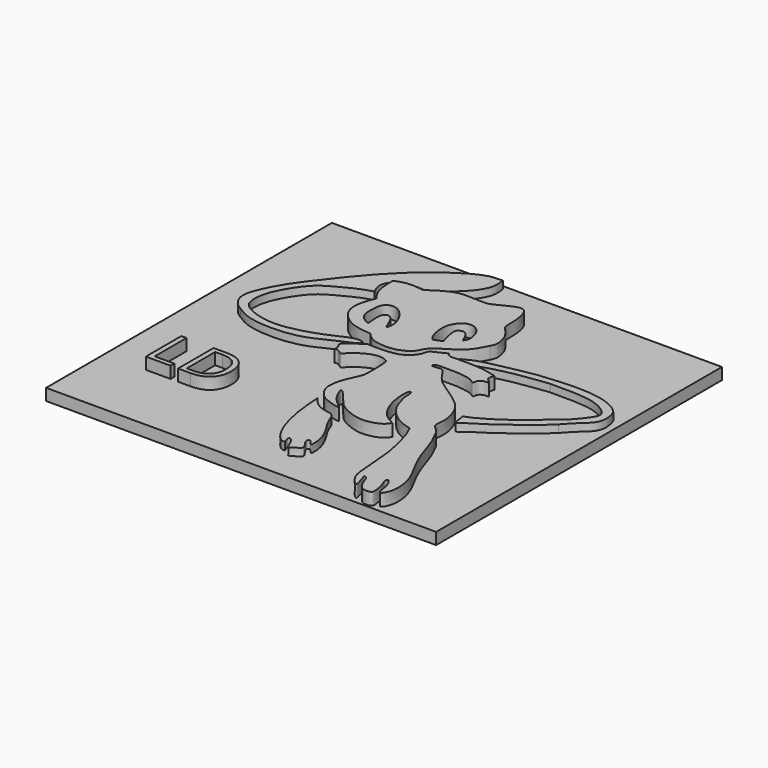
from build123d import *

# Parameters (mm, degrees)
F1_DEPTH     = 5.334
F2_DEPTH     = 3.302
F3_W         = 169.9430719018
F3_H         = 155.6462794542
F4_DEPTH     = 5.08
F5_DEPTH     = 5.08
F6_TEXT_SIZE = 27.0730789958
F7_DEPTH     = 5.08
F8_DEPTH     = 2.54


# Not quite as in the source:
# - Text() gives the source's letters only with a copy of the font that has no kerning and outlines rounded to 1/6400 em; it was checked with that copy


with BuildPart() as f1:
    # F0 (on Top) → F1 (new body)
    with BuildSketch(Plane.XY):
        with BuildLine():
            add(Edge.make_bspline(
                [(-36.8846021593, 36.0807068646), (-37.3919205691, 36.745355779), (-38.573167318, 38.2929329101), (-40.5014475338, 42.4143572996), (-40.7107590613, 48.2182279222), (-40.6138391704, 49.4369952817), (-40.5808985233, 49.8512238264)],
                knots=[0, 0, 0, 0, 0.2194056509, 0.5108669562, 0.8337559114, 1, 1, 1, 1], degree=3))
            add(Edge.make_bspline(
                [(-22.3644245416, 14.6438442171), (-24.6713467296, 14.8439032159), (-29.1783533156, 15.2347561151), (-34.882181479, 17.9727219406), (-39.1312315637, 23.0647945356), (-39.4935763136, 28.8302862551), (-37.8267011281, 33.815991482), (-37.1553457104, 35.4298653868), (-36.8846021593, 36.0807068646)],
                knots=[0, 0, 0, 0, 0.1893684443, 0.3699668893, 0.5515158216, 0.7238806595, 0.8886468645, 1, 1, 1, 1], degree=3))
            add(Edge.make_bspline(
                [(-5.2082133479, 12.2014991939), (-6.1207744444, 11.7172463933), (-8.3286563669, 10.545628396), (-15.353587418, 10.2966075507), (-19.699613734, 11.8971410348), (-21.5102479887, 13.7634179409), (-22.3644245416, 14.6438442171)],
                knots=[0, 0, 0, 0, 0.2165971456, 0.5240426358, 0.775464526, 1, 1, 1, 1], degree=3))
            add(Edge.make_bspline(
                [(15.1303568855, 32.9696908593), (14.5352451306, 31.8316959723), (13.2486953483, 29.3715075085), (10.2455123386, 24.8910940387), (3.5467707647, 21.2909451139), (-0.1632139181, 18.6569829706), (-1.6228436975, 15.6766034686), (-3.1877963332, 12.9531999529), (-4.5795045255, 12.4354117454), (-5.2082133479, 12.2014991939)],
                knots=[0, 0, 0, 0, 0.1407144931, 0.3042053849, 0.4994170574, 0.6491627195, 0.7763538673, 0.8989671128, 1, 1, 1, 1], degree=3))
            add(Edge.make_bspline(
                [(-28.5498145968, 50.8658960462), (-27.3946017427, 51.6630685406), (-24.9466228795, 53.3523342114), (-20.0833499164, 56.0652919109), (-16.3542778469, 56.9634408184), (-12.2867311767, 56.8716252918), (-6.9153223537, 56.7342359886), (-4.3946916269, 56.665054576), (1.0627636823, 59.6982249817), (4.5886739884, 61.236413898), (8.2470343675, 61.4891197316), (9.8575595266, 56.0097175618), (10.1904654801, 52.4142595185), (10.0843781414, 47.0754303269), (11.5893851176, 45.8127835913), (14.8613176101, 41.8496715208), (15.5576528197, 39.0147495294), (16.4135900587, 35.7580508966), (15.5545549064, 33.8914382347), (15.1303568855, 32.9696908593)],
                knots=[0, 0, 0, 0, 0.0621112649, 0.1316182234, 0.188871196, 0.2491962953, 0.3167553376, 0.3643401957, 0.436758445, 0.4967888689, 0.546791506, 0.6123099758, 0.6728165948, 0.7378250462, 0.7790399568, 0.8445049968, 0.8965058511, 0.9488938107, 1, 1, 1, 1], degree=3))
            add(Edge.make_bspline(
                [(-40.5808985233, 49.8512238264), (-39.7577733728, 50.1889108848), (-38.0437485114, 50.8920895121), (-34.9342862767, 51.5058179945), (-31.3792002355, 51.3783823788), (-29.458277106, 51.0304457679), (-28.5498145968, 50.8658960462)],
                knots=[0, 0, 0, 0, 0.234957575, 0.4892611102, 0.7584561682, 1, 1, 1, 1], degree=3))
        make_face()
        with BuildLine():
            add(Edge.make_bspline(
                [(-27.7441535145, 20.2597975731), (-27.836523165, 21.3377254697), (-28.0205851584, 23.4856772729), (-28.2064858053, 26.7533419634), (-27.3095138698, 28.5803581568), (-25.8242693753, 29.158776732), (-23.9397520395, 27.8647529376), (-22.7818146955, 25.7716562911), (-21.7167721967, 22.9536226595), (-21.1669852724, 21.9621876443), (-20.9360662848, 21.5457696468)],
                knots=[0, 0, 0, 0, 0.1498442019, 0.2985896596, 0.4110847443, 0.5056814579, 0.6233821967, 0.7537217582, 0.89655934, 1, 1, 1, 1], degree=3))
            add(Edge.make_bspline(
                [(-20.9360662848, 21.5457696468), (-20.6845803928, 22.4517973521), (-20.1286034759, 24.4548142458), (-21.2599441765, 28.7542103146), (-23.5058865444, 32.3709839432), (-26.9334066004, 35.3160516517), (-30.5123126311, 35.2735079139), (-32.7990191763, 33.0795235548), (-32.9444978647, 29.4825750713), (-33.2245472294, 25.7467879432), (-31.8503260445, 22.5933797005), (-29.5656235756, 20.8892744088), (-28.312173584, 20.4560980688), (-27.7441535145, 20.2597975731)],
                knots=[0, 0, 0, 0, 0.0851228406, 0.1881868366, 0.292340602, 0.3959368999, 0.4853122137, 0.5684365665, 0.6615536453, 0.7584972412, 0.8490847261, 0.9316104312, 1, 1, 1, 1], degree=3))
        make_face(mode=Mode.SUBTRACT)
        with BuildLine():
            add(Edge.make_bspline(
                [(5.4089953192, 30.3651615977), (4.9974793972, 31.3635089709), (4.2164206085, 33.2583760916), (2.492858238, 35.4574563274), (1.1828097347, 35.7536675932), (-1.0889632523, 34.9032052933), (-1.0761434624, 32.5663825666), (-0.7105408655, 30.3909840554), (-0.0619549295, 27.5454399373), (0.4242136144, 26.3185378529), (0.6415589014, 25.7700420916)],
                knots=[0, 0, 0, 0, 0.1500445323, 0.2847850944, 0.377641595, 0.497182947, 0.616278328, 0.7433829902, 0.8852774448, 1, 1, 1, 1], degree=3))
            Line((0.6415589014, 25.7700420916), (-3.0919760466, 24.3340656161))
            add(Edge.make_bspline(
                [(-3.0919760466, 24.3340656161), (-3.6746172439, 25.0952157056), (-4.9790959932, 26.7993590469), (-5.9269204187, 31.3877090281), (-5.8129309399, 36.1864843136), (-3.2806174064, 39.831657957), (-1.0494876922, 41.0503171402), (2.1831388461, 41.2713590695), (5.273039036, 38.380179271), (6.3476776556, 34.9097936113), (6.6819460197, 32.0494739818), (5.8108081984, 30.8968227282), (5.4089953192, 30.3651615977)],
                knots=[0, 0, 0, 0, 0.0943242152, 0.2111830315, 0.3310976043, 0.4422336843, 0.5274260332, 0.6207101402, 0.729021317, 0.8337202238, 0.9233033465, 1, 1, 1, 1], degree=3))
        make_face(mode=Mode.SUBTRACT)
    extrude(amount=F1_DEPTH)


with BuildPart() as f1b:
    # F0 (on Top) → F1, piece 2 (new body)
    with BuildSketch(Plane.XY):
        with BuildLine():
            add(Edge.make_bspline(
                [(30.0683174282, 16.6960265487), (27.7743567444, 17.2982553033), (22.996366427, 18.5526112206), (14.1217566151, 18.5069548483), (10.9595550033, 18.4055071495), (8.914888562, 18.2892193751), (8.1286790312, 19.3965578852), (7.7262688428, 19.9633333832)],
                knots=[0, 0, 0, 0, 0.2687230853, 0.5597115543, 0.7341470669, 0.8639269499, 1, 1, 1, 1], degree=3))
            add(Edge.make_bspline(
                [(7.7262688428, 19.9633333832), (6.7843841918, 19.4219987594), (4.8626373132, 18.3175024471), (0.9491517041, 16.983214183), (0.9172062675, 14.0816922981), (-1.1563972414, 11.1645043961), (-4.2681909188, 8.7975654115), (-10.2481427233, 7.7101704983), (-15.7637806819, 7.8784264398), (-17.5742383687, 7.9638167156), (-18.2920843363, 7.9976739362)],
                knots=[0, 0, 0, 0, 0.1189762035, 0.2427496271, 0.3446266716, 0.463365679, 0.5892044553, 0.7483578638, 0.9002239632, 1, 1, 1, 1], degree=3))
            add(Edge.make_bspline(
                [(-18.2920843363, 7.9976739362), (-19.2081909322, 7.3508545619), (-21.220968544, 5.9297278487), (-26.2844384077, 2.5837754081), (-25.5818429798, 1.1641009834), (-24.788360107, 0.7943681377), (-24.7400624967, -0.7928668879), (-24.7462409395, -1.4706101124), (-24.7490536422, -1.7791490536)],
                knots=[0, 0, 0, 0, 0.2335516694, 0.5131363244, 0.6318283516, 0.7367278182, 0.8801467617, 1, 1, 1, 1], degree=3))
            add(Edge.make_bspline(
                [(-24.7490536422, -1.7791490536), (-24.2594300604, -1.6489843167), (-23.1371940302, -1.3506417469), (-20.7418558435, -3.9319628807), (-19.8396284785, -1.3153314822), (-15.2791573927, 1.747858691), (-12.0049756273, 3.1979621252), (-8.2035408147, 3.7607412239), (-6.3214470372, 2.7044753683), (-5.4122591391, 2.1942222957)],
                knots=[0, 0, 0, 0, 0.1027998361, 0.2356211674, 0.3469371625, 0.5398555958, 0.7001501422, 0.8551507554, 1, 1, 1, 1], degree=3))
            add(Edge.make_bspline(
                [(-5.4122591391, -11.4604206756), (-5.2622117063, -11.0833952824), (-4.8483954868, -10.0435959346), (-4.8531432648, -5.796717989), (-4.8905091249, -0.455510217), (-5.2613557919, 1.4278523975), (-5.4122591391, 2.1942222957)],
                knots=[0, 0, 0, 0, 0.16298087, 0.4494853805, 0.7759869344, 1, 1, 1, 1], degree=3))
            add(Edge.make_bspline(
                [(-5.4122591391, -11.4604206756), (-5.7180365241, -12.1910633261), (-6.4589745929, -13.9615047682), (-8.7341618296, -18.823732403), (-9.3339817846, -22.6702412315), (-9.3862087635, -25.4827799286), (-8.6161951623, -27.2256408895), (-8.2267019898, -28.1072258949)],
                knots=[0, 0, 0, 0, 0.1760181488, 0.4265146922, 0.6415927054, 0.8187081449, 1, 1, 1, 1], degree=3))
            add(Edge.make_bspline(
                [(-8.2267019898, -28.1072258949), (-7.6234509095, -28.9847780463), (-6.3158368471, -30.886970303), (-3.3578440432, -33.0385452557), (4.7605685311, -35.3009211391), (0.7062696421, -32.348079143), (-2.6369370543, -28.938166705), (-4.7745965374, -23.008879984), (-2.1692361288, -25.4214104232), (0.0596427785, -28.1204059957), (3.5703763797, -32.828689266), (9.4441591128, -35.6788887604), (15.6783436568, -37.2193911759), (22.840726257, -35.0789922839), (24.1300062291, -32.9878270093), (24.6503651142, -32.1438238025)],
                knots=[0, 0, 0, 0, 0.0644771481, 0.1397614166, 0.2278212025, 0.2838940026, 0.3731896446, 0.4478304981, 0.4963143315, 0.5679076052, 0.6548180235, 0.7466462144, 0.8393730298, 0.9351702711, 1, 1, 1, 1], degree=3))
            add(Edge.make_bspline(
                [(24.6503651142, -32.1438238025), (22.7874017729, -31.1547850766), (18.978892069, -29.1328646762), (15.7565133464, -22.5588668197), (14.3110475227, -17.0219112758), (14.2258983476, -9.955668629), (16.1051306441, -10.5144580218), (15.6702473707, -13.747750159), (17.0855807883, -18.568062254), (18.3355817835, -22.1596484216), (21.6146077655, -26.502386498), (26.1560860605, -29.9186464967), (29.8500456849, -30.9730548373), (31.7023843527, -31.501788646)],
                knots=[0, 0, 0, 0, 0.1044502141, 0.213530586, 0.3203453584, 0.4213187613, 0.4580269744, 0.5290816996, 0.6236498562, 0.7054940824, 0.8011178875, 0.9002704239, 1, 1, 1, 1], degree=3))
            add(Edge.make_bspline(
                [(31.7023843527, -31.501788646), (32.4317515175, -33.0339186757), (34.0418847304, -36.4162116639), (35.891222752, -44.0199699231), (36.7066142268, -48.1595329342), (36.9354538826, -49.5206387254), (37.0256751776, -50.0572621822)],
                knots=[0, 0, 0, 0, 0.2736015544, 0.6039961368, 0.8438732953, 1, 1, 1, 1], degree=3))
            add(Edge.make_bspline(
                [(37.0256751776, -50.0572621822), (37.2529570378, -52.2585996466), (37.7295250837, -56.874397374), (38.1744288141, -65.147375762), (39.0614282703, -71.473936135), (43.7073747885, -75.9926535392), (43.0041439625, -73.1870722683), (42.5863736095, -71.2442159702), (41.2192631142, -68.0900104475), (43.2122596535, -69.062811459), (43.8660534195, -72.1091856839), (46.0001837404, -75.8667367907), (48.2415322815, -76.7510536361), (51.5666329574, -76.464046498), (51.0718324014, -73.597450229), (50.7537782092, -69.9651897279), (49.0133489818, -67.3461961901), (49.5300726584, -65.1991280143), (51.3610203699, -67.2721869465), (52.3453968623, -70.4529473283), (52.995619021, -76.2204950553), (56.059449066, -71.996615036), (56.1941191956, -64.2541648711), (53.057015864, -56.2370554706), (47.5422537848, -47.2864849217), (44.2428025956, -35.181683009), (42.4634124655, -31.9627538165), (41.779063642, -30.7247620076)],
                knots=[0, 0, 0, 0, 0.0515181447, 0.1080240258, 0.1600193281, 0.200966199, 0.2242692528, 0.2561913518, 0.2869292175, 0.3071601688, 0.3426397052, 0.3829711635, 0.4133879878, 0.44506026, 0.4747807776, 0.5132716918, 0.5483859123, 0.5705941331, 0.5969574393, 0.6366393869, 0.6760617143, 0.7097084145, 0.7649651301, 0.8224062602, 0.8873011559, 0.9566563172, 1, 1, 1, 1], degree=3))
            add(Edge.make_bspline(
                [(41.779063642, -30.7247620076), (41.220519955, -29.4131194944), (40.1405083976, -26.8769005623), (36.3496730282, -24.6391556022), (37.9091307315, -19.6176807334), (35.5635143336, -10.6479929739), (30.5388392719, -5.8669855098), (23.9637593307, -1.3236326178), (17.1210038146, 2.9501551711), (13.8645399549, 9.8095100123), (11.3218741684, 9.2331700055), (8.0189997491, 8.9048258219), (9.6884536448, 10.9398859033), (12.9400373278, 10.6519892488), (17.7385160156, 10.8919830294), (21.7909115084, 10.3524706804), (25.1173197763, 9.8387273821), (27.8544362389, 7.7039501469), (27.5140398783, 10.0552824679), (29.4509197324, 11.6524955754), (32.6539040013, 11.3234634506), (30.9452406108, 12.542717614), (30.0683174282, 13.1684653461)],
                knots=[0, 0, 0, 0, 0.0519267935, 0.1004067156, 0.1547860225, 0.2308120849, 0.2975658467, 0.3688932812, 0.4426002883, 0.5078563984, 0.5467057553, 0.5855180915, 0.6152135834, 0.6611250141, 0.7174470552, 0.7689076739, 0.8172224822, 0.8564603738, 0.8862383123, 0.9262880687, 0.962169435, 1, 1, 1, 1], degree=3))
            add(Edge.make_bspline(
                [(30.0683174282, 13.1684653461), (29.9041852058, 13.3684306238), (29.4381629957, 13.9361939752), (29.8205842702, 15.6110511778), (30.0683174282, 16.6960265487)],
                knots=[0, 0, 0, 0, 0.3521982834, 1, 1, 1, 1], degree=3))
        make_face()
    extrude(amount=F1_DEPTH)


with BuildPart() as f2:
    # F0 (on Top) → F2 (new body)
    with BuildSketch(Plane.XY):
        with BuildLine():
            add(Edge.make_bspline(
                [(-43.0377721786, 42.7853837609), (-43.4217519294, 43.5555106027), (-44.2704707094, 45.2577386818), (-44.7495303082, 49.6843935754), (-41.0137641329, 52.7815034964), (-36.6859509281, 54.4525017318), (-31.3441059726, 54.4142323895), (-29.2217337248, 54.0177284331), (-28.3044036478, 53.8463518023)],
                knots=[0, 0, 0, 0, 0.1383428068, 0.3057821096, 0.4812834692, 0.6632360629, 0.8544441539, 1, 1, 1, 1], degree=3))
            add(Edge.make_bspline(
                [(-28.3044036478, 53.8463518023), (-26.4073160355, 55.6555092544), (-22.6771829073, 59.2127504184), (-17.2353435255, 63.8393788129), (-13.8276032853, 69.6509731284), (-13.5447997553, 73.3805690433), (-13.8346112059, 75.3733824514), (-13.9714321122, 76.3141959906)],
                knots=[0, 0, 0, 0, 0.2399087284, 0.471718591, 0.6909669262, 0.8541045044, 1, 1, 1, 1], degree=3))
            add(Edge.make_bspline(
                [(-13.9714321122, 76.3141959906), (-15.6695767931, 76.3303285057), (-19.2883266624, 76.3647069291), (-25.3938334761, 73.7499379423), (-32.2227465198, 69.3257394868), (-37.0027510136, 65.6788461869), (-41.5089383745, 61.9702597728), (-43.2950078592, 60.2558688539), (-44.0782904625, 59.5040209591)],
                knots=[0, 0, 0, 0, 0.1571726677, 0.3349352838, 0.5326783847, 0.7051580212, 0.870696748, 1, 1, 1, 1], degree=3))
            add(Edge.make_bspline(
                [(-44.0782904625, 59.5040209591), (-46.5278412391, 57.082066591), (-52.097162839, 51.575488444), (-63.3309865981, 37.4942248425), (-71.4221468374, 26.4624379543), (-75.7339498561, 17.0106297705), (-76.6395144361, 11.8788318896), (-75.1074330935, 8.3160305556), (-73.204783322, 6.068043111), (-71.7088671371, 5.0905988199), (-70.9798410535, 4.6142470092)],
                knots=[0, 0, 0, 0, 0.1518529739, 0.3452543444, 0.517129726, 0.6613859031, 0.7623466126, 0.8489157512, 0.9263699669, 1, 1, 1, 1], degree=3))
            add(Edge.make_bspline(
                [(-70.9798410535, 4.6142470092), (-69.3666307118, 3.5770845145), (-65.6901376032, 1.2133997143), (-55.8893542983, -0.5183749), (-41.2432784113, 0.4464145968), (-31.0706871572, 6.483604405), (-24.0806480786, 8.8396956503), (-21.752412637, 11.3394508322), (-26.5347743619, 12.1529097756), (-32.3033005496, 9.1331545972), (-40.0565385081, 5.9205974959), (-50.0430210503, 3.1697487317), (-58.8129954214, 2.9178477888), (-66.9351159188, 5.4707126725), (-72.0186295298, 9.156570048), (-71.6690554507, 18.4329778003), (-66.5327096092, 27.8683616368), (-61.2862876559, 34.4220241119), (-54.7268271319, 37.7283730842), (-48.6744931046, 41.0395084453), (-44.8645902562, 42.2195589437), (-43.0377721786, 42.7853837609)],
                knots=[0, 0, 0, 0, 0.0465524502, 0.1060926513, 0.1790243597, 0.2452061951, 0.2968084881, 0.3232171179, 0.357646466, 0.4069920351, 0.4626730308, 0.5238603294, 0.5805035455, 0.6354123547, 0.6802029703, 0.7351769542, 0.7981924539, 0.8529702112, 0.9040331392, 0.9539846544, 1, 1, 1, 1], degree=3))
        make_face()
    extrude(amount=F2_DEPTH)


with BuildPart() as f2b:
    # F0 (on Top) → F2, piece 2 (new body)
    with BuildSketch(Plane.XY):
        with BuildLine():
            add(Edge.make_bspline(
                [(2.3568598554, -62.7967566252), (1.849591697, -62.7900183143), (0.4679465245, -62.7716651917), (-3.2310828631, -58.8113433278), (-6.7057614708, -50.0665204215), (-8.6370836456, -38.8411168477), (-8.9614558541, -33.2628901217), (-9.1090472415, -30.7247620076)],
                knots=[0, 0, 0, 0, 0.099509161, 0.2710328838, 0.51388907, 0.7788164808, 1, 1, 1, 1], degree=3))
            add(Edge.make_bspline(
                [(-9.1090472415, -30.7247620076), (-8.4235955574, -31.6189211927), (-6.9475052353, -33.5444540203), (-3.101528472, -36.1875069597), (1.8982272323, -36.366099626), (3.4405558722, -38.6877901024), (4.4761606927, -42.3593420867), (7.8964967826, -47.1650437774), (10.103858215, -52.0425869753), (10.7860608645, -55.6476684863), (10.6753618785, -57.5461375395), (10.9225050319, -59.3049638311), (9.4107167153, -57.6424469164), (8.5616404275, -56.4503239427), (7.5237963592, -56.8148042208), (7.6117730332, -58.1583165289), (8.9359028975, -60.1929547878), (10.1219675513, -61.7535687362), (9.4773292634, -62.9623853428), (7.0627564007, -64.3325582518), (5.4694748144, -65.4986569004), (4.5573424059, -62.78355908), (3.3761804254, -60.4551449839), (2.1377112045, -59.3756823228), (1.4345728768, -60.1256467658), (1.8841051195, -61.4401596052), (2.1958233582, -62.3346530955), (2.3568598554, -62.7967566252)],
                knots=[0, 0, 0, 0, 0.0496809561, 0.1069857733, 0.1646060762, 0.2058387605, 0.2571628324, 0.3222353289, 0.3845712685, 0.4346179158, 0.4726711954, 0.4992092936, 0.5325676268, 0.5654673868, 0.5880449987, 0.6160765379, 0.6586074123, 0.6943476006, 0.72222254, 0.7675356615, 0.7994953394, 0.8396297218, 0.8851573032, 0.9154600181, 0.9370908196, 0.9675005412, 1, 1, 1, 1], degree=3))
        make_face()
    extrude(amount=F2_DEPTH)


with BuildPart() as f2c:
    # F0 (on Top) → F2, piece 3 (new body)
    with BuildSketch(Plane.XY):
        with BuildLine():
            add(Edge.make_bspline(
                [(10.7216527686, 22.0162756741), (12.1246687267, 22.8148610446), (15.339687331, 24.6448237106), (23.6197362006, 26.4763189676), (32.72292454, 28.3516074967), (37.0192507628, 29.0816873989), (38.9400422573, 29.4080898166)],
                knots=[0, 0, 0, 0, 0.210423914, 0.4821875291, 0.7684976098, 1, 1, 1, 1], degree=3))
            add(Edge.make_bspline(
                [(10.7216527686, 22.0162756741), (11.0952281861, 21.6401005628), (11.9676852339, 20.7615721278), (15.1851161792, 20.2060896425), (20.1867499974, 22.1900920896), (27.3159099422, 24.2389696372), (36.615664636, 25.8884813304), (42.8756191809, 26.6520064029), (46.0081286728, 27.0340777934)],
                knots=[0, 0, 0, 0, 0.0904593315, 0.2112609063, 0.3729533578, 0.5659140772, 0.7827814461, 1, 1, 1, 1], degree=3))
            add(Edge.make_bspline(
                [(46.0081286728, 27.0340777934), (48.7258841079, 27.0612678355), (54.4256706903, 27.1182918912), (64.5466285691, 26.6819854244), (71.2784960569, 23.5683344076), (74.4956568823, 20.0928312055), (72.370302212, 16.1583995878), (68.2328509473, 10.8727360954), (63.0282482519, 6.6939099868), (60.288196872, 4.4211072069), (59.0115785599, 3.3621848561)],
                knots=[0, 0, 0, 0, 0.1437483771, 0.3014749084, 0.4359008913, 0.5332154076, 0.6294905174, 0.7592457502, 0.8878301019, 1, 1, 1, 1], degree=3))
            add(Edge.make_bspline(
                [(59.0115785599, 3.3621848561), (56.9423383347, 1.6375621217), (52.775286197, -1.8354966196), (46.5278179073, -6.1349616625), (39.331175356, -10.0891007633), (37.5946538004, -10.0778540145), (38.361869053, -11.9948167923), (38.4145231293, -16.8707660308), (41.9490027911, -13.083803004), (47.7757044759, -10.0981764978), (54.0702257822, -5.0810900312), (60.5319653238, -0.5910086566), (64.8441388463, 3.4273348996), (67.067630589, 5.4993187077)],
                knots=[0, 0, 0, 0, 0.1094389502, 0.2203890133, 0.3295663194, 0.369726266, 0.4213415268, 0.4936271411, 0.5627007536, 0.6656686645, 0.7754420094, 0.884210866, 1, 1, 1, 1], degree=3))
            add(Edge.make_bspline(
                [(67.067630589, 5.4993187077), (68.4073962182, 7.0026565142), (71.2661439341, 10.3161375403), (78.3602736598, 15.59597471), (76.7631828785, 22.33495377), (75.9328380227, 24.1133533418)],
                knots=[0, 0, 0, 0, 0.3098887474, 0.6604961476, 1, 1, 1, 1], degree=3))
            add(Edge.make_bspline(
                [(38.9400422573, 29.4080898166), (42.1234440462, 29.7199891996), (48.5724313187, 30.3518400576), (58.6475201749, 30.6661036157), (67.9584350083, 29.3917039016), (73.8641097497, 26.3531807622), (75.3402605954, 24.7549413105), (75.9328380227, 24.1133533418)],
                knots=[0, 0, 0, 0, 0.2286564396, 0.4632159453, 0.6902384315, 0.8756511139, 1, 1, 1, 1], degree=3))
        make_face()
    extrude(amount=F2_DEPTH)


with BuildPart() as f4:
    # F3 (on face) → F4 (new body)
    with BuildSketch(Plane(origin=(0, 0, 0), x_dir=(1, 0, 0), z_dir=(0, 0, -1))):
        with Locations((-4.9392692745, -0.3463253379)):
            Rectangle(F3_W, F3_H)
        with BuildLine():
            add(Edge.make_bspline(
                [(30.0683174282, -13.1684653461), (29.9041852058, -13.3684306238), (29.4381629957, -13.9361939752), (29.8205842702, -15.6110511778), (30.0683174282, -16.6960265487)],
                knots=[0, 0, 0, 0, 0.3521982834, 1, 1, 1, 1], degree=3))
            add(Edge.make_bspline(
                [(30.0683174282, -16.6960265487), (27.7743567444, -17.2982553033), (22.996366427, -18.5526112206), (14.1217566151, -18.5069548483), (10.9595550033, -18.4055071495), (8.914888562, -18.2892193751), (8.1286790312, -19.3965578852), (7.7262688428, -19.9633333832)],
                knots=[0, 0, 0, 0, 0.2687230853, 0.5597115543, 0.7341470669, 0.8639269499, 1, 1, 1, 1], degree=3))
            add(Edge.make_bspline(
                [(7.7262688428, -19.9633333832), (6.7843841918, -19.4219987594), (4.8626373132, -18.3175024471), (0.9491517041, -16.983214183), (0.9172062675, -14.0816922981), (-1.1563972414, -11.1645043961), (-4.2681909188, -8.7975654115), (-10.2481427233, -7.7101704983), (-15.7637806819, -7.8784264398), (-17.5742383687, -7.9638167156), (-18.2920843363, -7.9976739362)],
                knots=[0, 0, 0, 0, 0.1189762035, 0.2427496271, 0.3446266716, 0.463365679, 0.5892044553, 0.7483578638, 0.9002239632, 1, 1, 1, 1], degree=3))
            add(Edge.make_bspline(
                [(-18.2920843363, -7.9976739362), (-19.2081909322, -7.3508545619), (-21.220968544, -5.9297278487), (-26.2844384077, -2.5837754081), (-25.5818429798, -1.1641009834), (-24.788360107, -0.7943681377), (-24.7400624967, 0.7928668879), (-24.7462409395, 1.4706101124), (-24.7490536422, 1.7791490536)],
                knots=[0, 0, 0, 0, 0.2335516694, 0.5131363244, 0.6318283516, 0.7367278182, 0.8801467617, 1, 1, 1, 1], degree=3))
            add(Edge.make_bspline(
                [(-24.7490536422, 1.7791490536), (-24.2594300604, 1.6489843167), (-23.1371940302, 1.3506417469), (-20.7418558435, 3.9319628807), (-19.8396284785, 1.3153314822), (-15.2791573927, -1.747858691), (-12.0049756273, -3.1979621252), (-8.2035408147, -3.7607412239), (-6.3214470372, -2.7044753683), (-5.4122591391, -2.1942222957)],
                knots=[0, 0, 0, 0, 0.1027998361, 0.2356211674, 0.3469371625, 0.5398555958, 0.7001501422, 0.8551507554, 1, 1, 1, 1], degree=3))
            add(Edge.make_bspline(
                [(-5.4122591391, 11.4604206756), (-5.2622117063, 11.0833952824), (-4.8483954868, 10.0435959346), (-4.8531432648, 5.796717989), (-4.8905091249, 0.455510217), (-5.2613557919, -1.4278523975), (-5.4122591391, -2.1942222957)],
                knots=[0, 0, 0, 0, 0.16298087, 0.4494853805, 0.7759869344, 1, 1, 1, 1], degree=3))
            add(Edge.make_bspline(
                [(-5.4122591391, 11.4604206756), (-5.7180365241, 12.1910633261), (-6.4589745929, 13.9615047682), (-8.7341618296, 18.823732403), (-9.3339817846, 22.6702412315), (-9.3862087635, 25.4827799286), (-8.6161951623, 27.2256408895), (-8.2267019898, 28.1072258949)],
                knots=[0, 0, 0, 0, 0.1760181488, 0.4265146922, 0.6415927054, 0.8187081449, 1, 1, 1, 1], degree=3))
            add(Edge.make_bspline(
                [(-8.2267019898, 28.1072258949), (-7.6234509095, 28.9847780463), (-6.3158368471, 30.886970303), (-3.3578440432, 33.0385452557), (4.7605685311, 35.3009211391), (0.7062696421, 32.348079143), (-2.6369370543, 28.938166705), (-4.7745965374, 23.008879984), (-2.1692361288, 25.4214104232), (0.0596427785, 28.1204059957), (3.5703763797, 32.828689266), (9.4441591128, 35.6788887604), (15.6783436568, 37.2193911759), (22.840726257, 35.0789922839), (24.1300062291, 32.9878270093), (24.6503651142, 32.1438238025)],
                knots=[0, 0, 0, 0, 0.0644771481, 0.1397614166, 0.2278212025, 0.2838940026, 0.3731896446, 0.4478304981, 0.4963143315, 0.5679076052, 0.6548180235, 0.7466462144, 0.8393730298, 0.9351702711, 1, 1, 1, 1], degree=3))
            add(Edge.make_bspline(
                [(24.6503651142, 32.1438238025), (22.7874017729, 31.1547850766), (18.978892069, 29.1328646762), (15.7565133464, 22.5588668197), (14.3110475227, 17.0219112758), (14.2258983476, 9.955668629), (16.1051306441, 10.5144580218), (15.6702473707, 13.747750159), (17.0855807883, 18.568062254), (18.3355817835, 22.1596484216), (21.6146077655, 26.502386498), (26.1560860605, 29.9186464967), (29.8500456849, 30.9730548373), (31.7023843527, 31.501788646)],
                knots=[0, 0, 0, 0, 0.1044502141, 0.213530586, 0.3203453584, 0.4213187613, 0.4580269744, 0.5290816996, 0.6236498562, 0.7054940824, 0.8011178875, 0.9002704239, 1, 1, 1, 1], degree=3))
            add(Edge.make_bspline(
                [(31.7023843527, 31.501788646), (32.4317515175, 33.0339186757), (34.0418847304, 36.4162116639), (35.891222752, 44.0199699231), (36.7066142268, 48.1595329342), (36.9354538826, 49.5206387254), (37.0256751776, 50.0572621822)],
                knots=[0, 0, 0, 0, 0.2736015544, 0.6039961368, 0.8438732953, 1, 1, 1, 1], degree=3))
            add(Edge.make_bspline(
                [(37.0256751776, 50.0572621822), (37.2529570378, 52.2585996466), (37.7295250837, 56.874397374), (38.1744288141, 65.147375762), (39.0614282703, 71.473936135), (43.7073747885, 75.9926535392), (43.0041439625, 73.1870722683), (42.5863736095, 71.2442159702), (41.2192631142, 68.0900104475), (43.2122596535, 69.062811459), (43.8660534195, 72.1091856839), (46.0001837404, 75.8667367907), (48.2415322815, 76.7510536361), (51.5666329574, 76.464046498), (51.0718324014, 73.597450229), (50.7537782092, 69.9651897279), (49.0133489818, 67.3461961901), (49.5300726584, 65.1991280143), (51.3610203699, 67.2721869465), (52.3453968623, 70.4529473283), (52.995619021, 76.2204950553), (56.059449066, 71.996615036), (56.1941191956, 64.2541648711), (53.057015864, 56.2370554706), (47.5422537848, 47.2864849217), (44.2428025956, 35.181683009), (42.4634124655, 31.9627538165), (41.779063642, 30.7247620076)],
                knots=[0, 0, 0, 0, 0.0515181447, 0.1080240258, 0.1600193281, 0.200966199, 0.2242692528, 0.2561913518, 0.2869292175, 0.3071601688, 0.3426397052, 0.3829711635, 0.4133879878, 0.44506026, 0.4747807776, 0.5132716918, 0.5483859123, 0.5705941331, 0.5969574393, 0.6366393869, 0.6760617143, 0.7097084145, 0.7649651301, 0.8224062602, 0.8873011559, 0.9566563172, 1, 1, 1, 1], degree=3))
            add(Edge.make_bspline(
                [(41.779063642, 30.7247620076), (41.220519955, 29.4131194944), (40.1405083976, 26.8769005623), (36.3496730282, 24.6391556022), (37.9091307315, 19.6176807334), (35.5635143336, 10.6479929739), (30.5388392719, 5.8669855098), (23.9637593307, 1.3236326178), (17.1210038146, -2.9501551711), (13.8645399549, -9.8095100123), (11.3218741684, -9.2331700055), (8.0189997491, -8.9048258219), (9.6884536448, -10.9398859033), (12.9400373278, -10.6519892488), (17.7385160156, -10.8919830294), (21.7909115084, -10.3524706804), (25.1173197763, -9.8387273821), (27.8544362389, -7.7039501469), (27.5140398783, -10.0552824679), (29.4509197324, -11.6524955754), (32.6539040013, -11.3234634506), (30.9452406108, -12.542717614), (30.0683174282, -13.1684653461)],
                knots=[0, 0, 0, 0, 0.0519267935, 0.1004067156, 0.1547860225, 0.2308120849, 0.2975658467, 0.3688932812, 0.4426002883, 0.5078563984, 0.5467057553, 0.5855180915, 0.6152135834, 0.6611250141, 0.7174470552, 0.7689076739, 0.8172224822, 0.8564603738, 0.8862383123, 0.9262880687, 0.962169435, 1, 1, 1, 1], degree=3))
        make_face(mode=Mode.SUBTRACT)
    extrude(amount=F4_DEPTH)

    # F6 (on face) → F7 (join)
    with BuildSketch(Plane.XY):
        with Locations((-74.3471160531, -45.9343194962)):
            Text('LD', F6_TEXT_SIZE, font='Open Sans', text_align=(TextAlign.LEFT, TextAlign.BOTTOM))
    extrude(amount=F7_DEPTH)

    # F6 (on face) → F8 (join)
    with BuildSketch(Plane.XY):
        with Locations((-74.3471160531, -45.9343194962)):
            Text('LD', F6_TEXT_SIZE, font='Open Sans', text_align=(TextAlign.LEFT, TextAlign.BOTTOM))
    extrude(amount=F8_DEPTH)


with BuildPart() as f5:
    # F5 (new): a face of the model
    f5_faces = [f1b.part.faces().sort_by_distance(p)[0] for p in [
        (18.9065912912, -20.1747019139, 0),
    ]]
    extrude(f5_faces, amount=F5_DEPTH)


solid = Compound([f1.part, f1b.part, f2.part, f2b.part, f2c.part, f4.part, f5.part])
